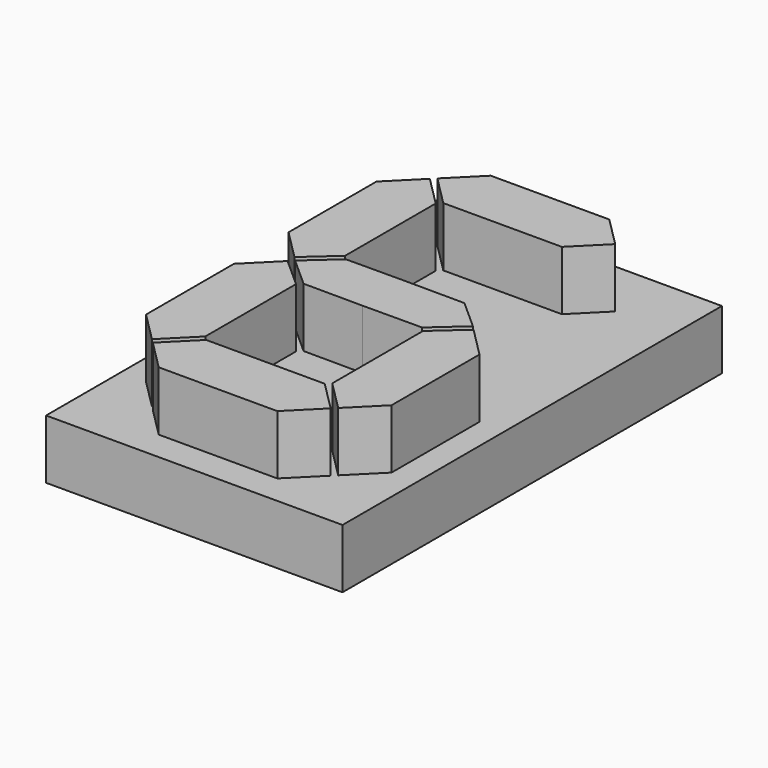
from build123d import *

# Parameters (mm, degrees)
F0_W     = 10
F0_H     = 16
F1_DEPTH = 2
F3_DEPTH = 2


# Not quite as in the source:
# - ends of sketch curves that miss each other by under 0.0002 mm in the source are joined


with BuildPart() as f1:
    # F0 (on Top) → F1 (new body)
    with BuildSketch(Plane.XY):
        Rectangle(F0_W, F0_H)
    extrude(amount=F1_DEPTH)

    # F2 (on face) → F3 (join)
    with BuildSketch(Plane.XY.offset(2)):
        Polygon((0, 7), (-2, 7), (-3, 6), (-2, 5), (0, 5), (2, 5), (3, 6), (2, 7), align=None)
        Polygon((-2.1414213562, 4.8585786438), (-3.1414213562, 5.8585786438), (-4.1414213562, 4.8585786438), (-4.1414213562, 1.1507223826), (-3.1374518146, 0.1453992321), (-2.1414213562, 1.0335195075), align=None)
        Polygon((2, 0.891659756), (2.00782e-05, 0.9006214721), (-2, 0.891659756), (-3, 0), (-2, -0.891659756), (-2.00782e-05, -0.9006214721), (2, -0.891659756), (3, 0), align=None)
        Polygon((0, -5), (-2, -5), (-3, -6), (-2, -7), (0, -7), (2, -7), (3, -6), (2, -5), align=None)
        Polygon((-4.1414213562, -4.8585786438), (-3.1414213562, -5.8585786438), (-2.1414213562, -4.8585786438), (-2.1414213562, -1.0335195075), (-3.1374518146, -0.1453992321), (-4.1414213562, -1.1507223826), align=None)
        Polygon((3.1374518146, -0.1453992321), (2.1414213562, -1.0335195075), (2.1414213562, -4.8585786438), (3.1414213562, -5.8585786438), (4.1414213562, -4.8585786438), (4.1414213562, -1.1507223826), align=None)
    extrude(amount=F3_DEPTH)


solid = f1.part
